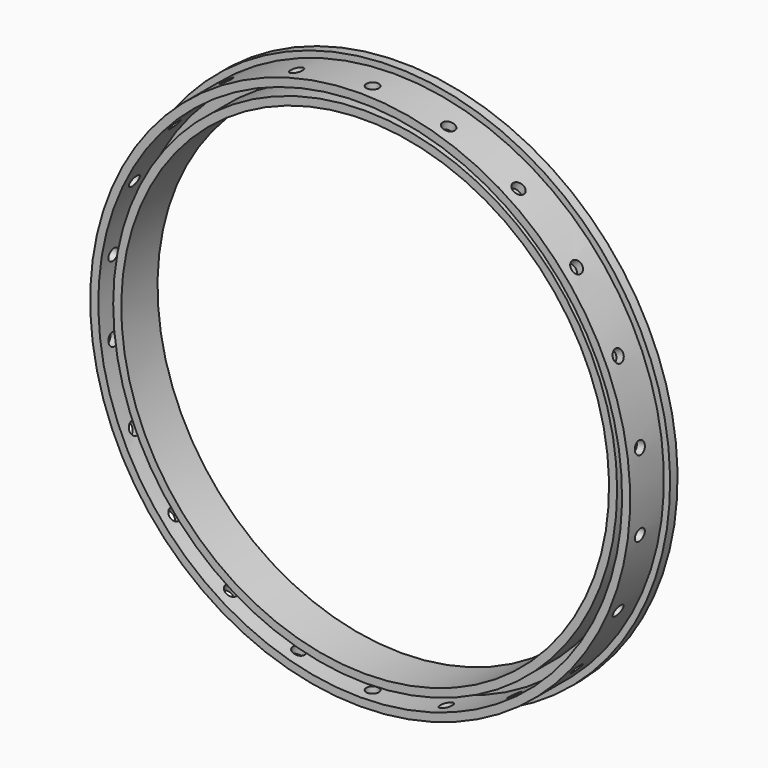
from build123d import *

# Parameters (mm, degrees)
F4_D            = 2
F4_DEPTH        = 2.2
F4_START        = 0.5114959
F4_TIP          = 0.600860619
F4_COPIES_COUNT = 22


# Not quite as in the source:
# - a pattern or mirror of a feature is missing from the dataset's text; its kind, count and spacing are read off the source's solid


with BuildPart() as f1:
    # F0 (on Right) → F1 (revolve)
    with BuildSketch(Plane.YZ):
        Polygon((0, -44.5), (0, -39.3), (-7.2982744314, -39.3), (-7.2982744314, -40.6), (-2.3, -40.6), (-2.3, -42.2), (-8.3, -42.2), (-8.3, -43.5), (-1.5, -43.5), (-1.5, -44.5), align=None)
    revolve(axis=Axis((0, 3.0112779704, 0), (0, 1, 0)))

    # F4
    # its depths count from where the whole tool has entered the part; down to there all is cleared
    with Locations(Plane.XY.offset(44).offset(-F4_START)):
        with Locations((0, -5.8)):
            f4 = Hole(F4_D / 2, depth=F4_DEPTH)
            with Locations((0, 0, -(F4_DEPTH + F4_TIP / 2))):  # 118° drill point
                Cone(0, F4_D / 2, F4_TIP, mode=Mode.SUBTRACT)

    # F4_copies: F4 ×22 about axis
    f4_copies_axis = Axis((0, 0, 0), (0, 1, 0))
    for i in range(1, F4_COPIES_COUNT):
        add(f4.rotate(f4_copies_axis, i * 360 / F4_COPIES_COUNT), mode=Mode.SUBTRACT)


solid = f1.part
